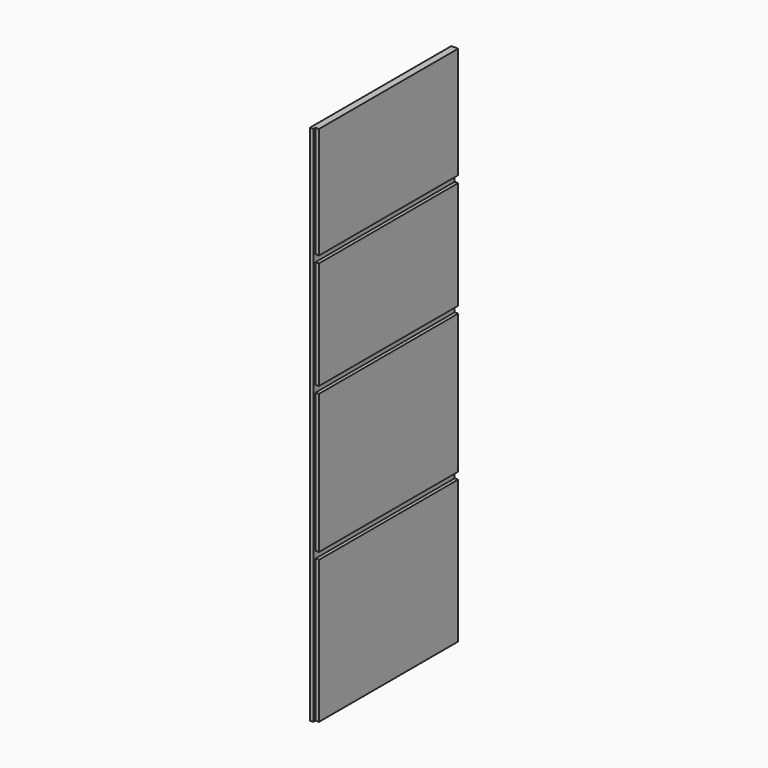
from build123d import *

# Parameters (mm, degrees)
F1_DEPTH = 406.35
F2_W     = 7.94
F2_H     = 6.35
F3_DEPTH = 1200.001


# Not quite as in the source:
# - a feature names something its author has since deleted; it is built from what else it names


with BuildPart() as f1:
    # F0 (on Front) → F1 (new body)
    with BuildSketch(Plane.XZ):
        Polygon((-29.5198056847, 967.7915206528), (-45.3948056847, 967.7915206528), (-45.3948056847, -232.2084793472), (-29.5198056847, -232.2084793472), (-29.5198056847, 95.7315206528), (-37.4598056847, 95.7315206528), (-37.4598056847, 111.6065206528), (-29.5198056847, 111.6065206528), (-29.5198056847, 431.6065206528), (-37.4598056847, 431.6065206528), (-37.4598056847, 447.4815206528), (-29.5198056847, 447.4815206528), (-29.5198056847, 695.7315206528), (-37.4598056847, 695.7315206528), (-37.4598056847, 711.6065206528), (-29.5198056847, 711.6065206528), align=None)
    extrude(amount=F1_DEPTH)

    # F2 (on face) → F3 (cut, through all)
    with BuildSketch(Plane.XY.offset(967.7915206528)):
        with Locations((-33.4898056847, -403.175)):
            Rectangle(F2_W, F2_H)
    extrude(amount=-F3_DEPTH, mode=Mode.SUBTRACT)


solid = f1.part
